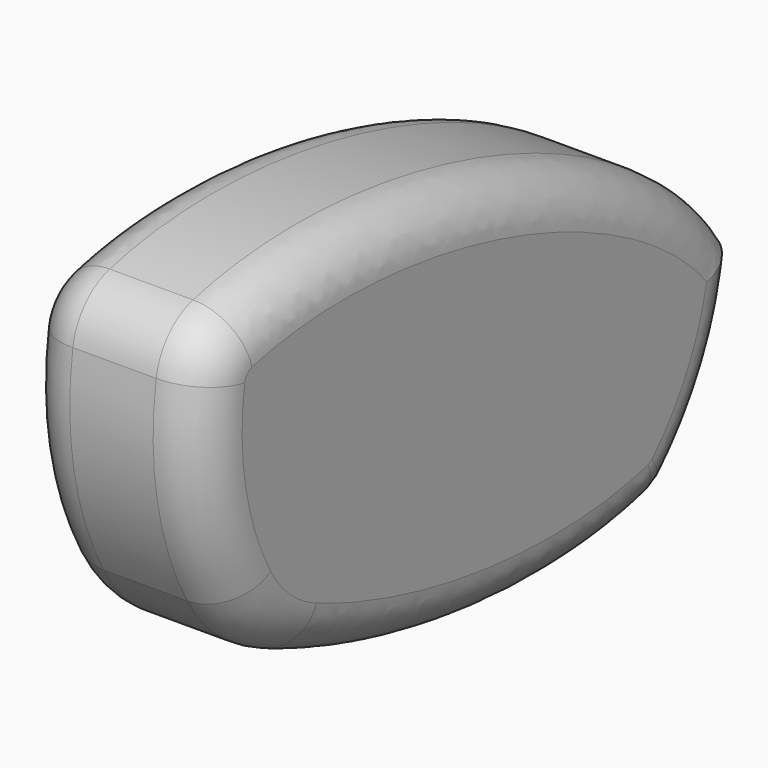
from build123d import *

# Parameters (mm, degrees)
F3_R = 5.08


with BuildPart() as f2:
    # F2: sweep along a path in F1
    with BuildLine(Plane.XZ) as f2_path:
        Line((-18.7538489699, 37.0099879801), (-37.481315434, 37.0099879801))
    # F0 (on Right) → F2 (sweep)
    with BuildSketch(Plane.YZ):
        with BuildLine():
            ThreePointArc((-63.2333904502, 21.6500088574), (-59.7109744357, 17.267735227), (-54.9707940163, 14.2440906808))
            add(Edge.make_bspline(
                [(-54.9707940163, 14.2440906808), (-29.557007786, 3.354277996), (-8.4298012229, 9.3640714915)],
                knots=[4.3330950452, 4.3330950452, 4.3330950452, 5.560977455, 5.560977455, 5.560977455], degree=2, weights=[1, 0.8173838698, 1]))
            Line((-8.4298012229, 9.3640714915), (-6.8284584686, 10.2392208894))
            ThreePointArc((-6.8284584686, 10.2392208894), (-0.5664539631, 18.7231469313), (2.5196485221, 28.8060866296))
            add(Edge.make_bspline(
                [(2.5196485221, 28.8060866296), (-16.9083238195, 60.0320255806), (-62.463944192, 48.5690009646)],
                knots=[0.4350349648, 0.4350349648, 0.4350349648, 2.3821123688, 2.3821123688, 2.3821123688], degree=2, weights=[1, 0.5623769731, 1]))
            ThreePointArc((-62.463944192, 48.5690009646), (-65.6073437062, 46.688684411), (-67.1892597454, 43.38503605))
            ThreePointArc((-67.1892597454, 43.38503605), (-67.0434822848, 32.1840618928), (-63.2333904502, 21.6500088574))
        make_face()
    sweep(path=f2_path.line)

    # F3
    f3_edges = [f2.edges().sort_by_distance(p)[0] for p in [
        (-18.727466, -67.043482, 32.184062),
        (-18.727466, -59.710974, 17.267735),
        (-18.727466, -32.047448, 8.151815),
        (-18.727466, -7.62913, 9.801646),
        (-18.727466, -0.566454, 18.723147),
        (-18.727466, -27.276683, 46.954007),
        (-18.727466, -65.607344, 46.688684),
        (0, -67.043482, 32.184062),
        (0, -59.710974, 17.267735),
        (0, -30.736335, 8.00371),
        (0, -7.62913, 9.801646),
        (0, -0.566454, 18.723147),
        (0, -25.26983, 46.370482),
        (0, -65.607344, 46.688684),
    ]]
    fillet(f3_edges, radius=F3_R)


solid = f2.part
